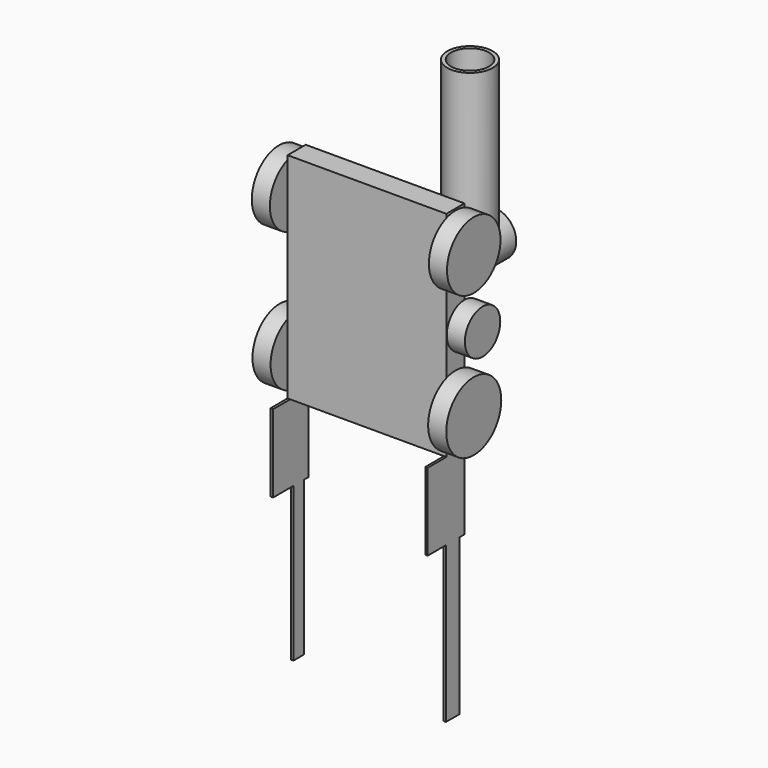
from build123d import *

# Parameters (mm, degrees)
F0_W      = 89.10818398
F0_H      = 120.1675757766
F1_DEPTH  = 12.7
F2_R      = 19.05
F3_DEPTH  = 10.16
F4_R      = 19.05
F5_DEPTH  = 10.16
F6_R      = 18.7667167596
F7_DEPTH  = 10.16
F8_R      = 19.2986234131
F9_DEPTH  = 10.16
F10_R     = 12.4156573735
F11_DEPTH = 10.16
F12_R     = 12.6694142054
F13_DEPTH = 76.2
F14_R     = 12.7449680287
F15_DEPTH = 92.456
F16_R     = 10.4865516495
F17_DEPTH = 76.2
F18_R     = 10.6677127508
F19_DEPTH = 88.9
F20_R     = 11.5560475943
F21_DEPTH = 25.4
F24_W     = 1.3282671571
F24_H     = 25.8222837001
F25_DEPTH = 43.434
F26_W     = 1.4417506754
F26_H     = 24.6515385807
F27_DEPTH = 43.688
F22_W     = 1.255504787
F22_H     = 24.4307331741
F30_DEPTH = 18.034
F23_W     = 1.2999391183
F23_H     = 24.1094622761
F31_DEPTH = 18.034
F36_W     = 1.3282671571
F36_H     = 9.5440435689
F37_DEPTH = 87.376
F38_W     = 1.4417506754
F38_H     = 7.3205276858
F39_DEPTH = 86.36


# Not quite as in the source:
# - the program builds the solid bodies; features that only make, move or delete a surface that nothing else refers to are left out


with BuildPart() as f1:
    # F0 (on Front) → F1 (new body)
    with BuildSketch(Plane.XZ):
        Rectangle(F0_W, F0_H)
    extrude(amount=F1_DEPTH)

    # F2 (on face) → F3 (join)
    with BuildSketch(Plane(origin=(-44.55409199, 0, 0), x_dir=(0, -1, 0), z_dir=(-1, 0, 0))):
        with Locations((6.0873422772, 39.9295948446)):
            Circle(F2_R)
    extrude(amount=F3_DEPTH)

    # F4 (on face) → F5 (join)
    with BuildSketch(Plane(origin=(-44.55409199, 0, 0), x_dir=(0, -1, 0), z_dir=(-1, 0, 0))):
        with Locations((5.5960081518, -38.5527424514)):
            Circle(F4_R)
    extrude(amount=F5_DEPTH)

    # F6 (on face) → F7 (join)
    with BuildSketch(Plane.YZ.offset(44.55409199)):
        with Locations((-6.1870645732, 40.3565391898)):
            Circle(F6_R)
    extrude(amount=F7_DEPTH)

    # F8 (on face) → F9 (join)
    with BuildSketch(Plane.YZ.offset(44.55409199)):
        with Locations((-6.1870645732, -39.2316170037)):
            Circle(F8_R)
    extrude(amount=F9_DEPTH)

    # F10 (on face) → F11 (join)
    with BuildSketch(Plane.YZ.offset(44.55409199)):
        Circle(F10_R)
    extrude(amount=F11_DEPTH)

    # F12 (on face) → F13 (join)
    with BuildSketch(Plane(origin=(0, 0, 0), x_dir=(-1, 0, 0), z_dir=(0, 1, 0))):
        Circle(F12_R)
    extrude(amount=F13_DEPTH)

    # F14 (on Top) → F15 (join)
    with BuildSketch(Plane.XY):
        with Locations((0, 59.6004612744)):
            Circle(F14_R)
    extrude(amount=F15_DEPTH)

    # F16 (on face) → F17 (cut)
    with BuildSketch(Plane(origin=(0, 76.2, 0), x_dir=(-1, 0, 0), z_dir=(0, 1, 0))):
        Circle(F16_R)
    extrude(amount=-F17_DEPTH, mode=Mode.SUBTRACT)

    # F18 (on face) → F19 (cut)
    with BuildSketch(Plane.XY.offset(92.456)):
        with Locations((0, 59.6004612744)):
            Circle(F18_R)
    extrude(amount=-F19_DEPTH, mode=Mode.SUBTRACT)

    # F20 (on Top) → F21 (cut)
    with BuildSketch(Plane.XY):
        with Locations((0, 12.4179841951)):
            Circle(F20_R)
    extrude(amount=-F21_DEPTH, mode=Mode.SUBTRACT)

    # F24 (on face) → F25 (join)
    with BuildSketch(Plane(origin=(0, 0, -60.0837878883), x_dir=(1, 0, 0), z_dir=(0, 0, -1))):
        with Locations((43.8899584115, 12.9111418501)):
            Rectangle(F24_W, F24_H)
    extrude(amount=F25_DEPTH)

    # F26 (on face) → F27 (join)
    with BuildSketch(Plane(origin=(0, 0, -60.0837878883), x_dir=(1, 0, 0), z_dir=(0, 0, -1))):
        with Locations((-43.8332166523, 12.3257692903)):
            Rectangle(F26_W, F26_H)
    extrude(amount=F27_DEPTH)

    # F22 (on Top) → F30 (join)
    with BuildSketch(Plane.XY):
        with Locations((14.0256239101, 12.215366587)):
            Rectangle(F22_W, F22_H)
    extrude(amount=-F30_DEPTH)

    # F23 (on Top) → F31 (join)
    with BuildSketch(Plane.XY):
        with Locations((-13.2890497334, 12.0547311381)):
            Rectangle(F23_W, F23_H)
    extrude(amount=-F31_DEPTH)

    # F36 (on face) → F37 (join)
    with BuildSketch(Plane(origin=(0, 0, -103.5177878883), x_dir=(1, 0, 0), z_dir=(0, 0, -1))):
        with Locations((43.8899584115, 8.1391200656)):
            Rectangle(F36_W, F36_H)
    extrude(amount=F37_DEPTH)

    # F38 (on face) → F39 (join)
    with BuildSketch(Plane(origin=(0, 0, -103.7717878883), x_dir=(1, 0, 0), z_dir=(0, 0, -1))):
        with Locations((-43.8332166523, 6.7722700769)):
            Rectangle(F38_W, F38_H)
    extrude(amount=F39_DEPTH)


solid = f1.part
